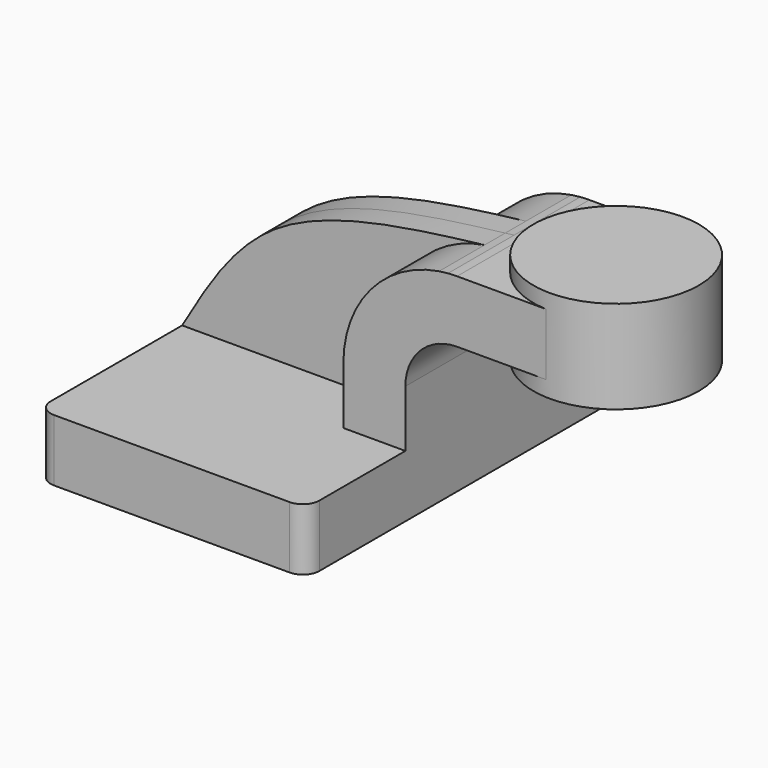
from build123d import *

# Parameters (mm, degrees)
F1_DEPTH = 63.5
F2_DEPTH = 25.4
F0_W     = 25.4
F0_H     = 19.05
F4_DEPTH = 25.4
F5_DEPTH = 7.9375
F7_R     = 5.08


# Not quite as in the source:
# - a feature names something its author has since deleted; it is built from what else it names


with BuildPart() as f1:
    # F0 (on Front) → F1 (new body, symmetric)
    with BuildSketch(Plane.XZ):
        Polygon((41.275, -9.525), (41.275, 9.525), (22.225, 9.525), (-41.275, 9.525), (-41.275, -9.525), align=None)
    extrude(amount=F1_DEPTH, both=True)

    # F0 (on Front) → F2 (join, symmetric)
    with BuildSketch(Plane.XZ):
        with BuildLine():
            Line((22.225, 9.525), (41.275, 9.525))
            Line((41.275, 9.525), (41.275, 27.0002))
            ThreePointArc((41.275, 27.0002), (45.9246798487, 38.2255201513), (57.15, 42.8752))
            Line((57.15, 42.8752), (60.325, 42.8752))
            Line((60.325, 42.8752), (60.325, 61.9252))
            Line((60.325, 61.9252), (57.15, 61.9252))
            ThreePointArc((57.15, 61.9252), (55.7573840511, 61.8974240417), (54.3669832056, 61.8141403475))
            add(Edge.make_bspline(
                [(51.6315731061, 61.4864666813), (52.5431025701, 61.5959254015), (53.4550436694, 61.7050265498), (54.3669832056, 61.8141403475)],
                knots=[0.9798743177, 0.9798743177, 0.9798743177, 0.9798743177, 1, 1, 1, 1], degree=3))
            ThreePointArc((51.6315731061, 61.4864666813), (30.5747607323, 49.6610094045), (22.225, 27.0002))
            Line((22.225, 27.0002), (22.225, 9.525))
        make_face()
    extrude(amount=F2_DEPTH, both=True)

    # F0 (on Front) → F4 (join, symmetric)
    with BuildSketch(Plane.XZ):
        with Locations((73.025, 52.4002)):
            Rectangle(F0_W, F0_H)
    extrude(amount=F4_DEPTH, both=True)

    # F0 (on Front) → F5 (join, symmetric)
    with BuildSketch(Plane.XZ):
        with BuildLine():
            Line((-41.275, 9.525), (22.225, 9.525))
            Line((22.225, 9.525), (22.225, 27.0002))
            ThreePointArc((22.225, 27.0002), (30.5747607323, 49.6610094045), (51.6315731061, 61.4864666813))
            add(Edge.make_bspline(
                [(-41.275, 9.525), (-33.3226171476, 23.2066083148), (-16.1059236769, 52.8331960278), (27.7493063598, 58.6186248213), (51.6315731061, 61.4864666813)],
                knots=[0, 0, 0, 0, 0.4525771396, 0.9798743177, 0.9798743177, 0.9798743177, 0.9798743177], degree=3))
        make_face()
    extrude(amount=F5_DEPTH, both=True)

    # F0 (on Front) → F6 (revolve)
    with BuildSketch(Plane.XZ):
        Polygon((85.725, 61.9252), (85.725, 42.8752), (85.725, 38.1), (111.125, 38.1), (111.125, 66.675), (85.725, 66.675), align=None)
    revolve(axis=Axis((85.6968834996, 0, 52.5015871972), (0, 0, -1)))

    # F7
    f7_edges = [f1.edges().sort_by_distance(p)[0] for p in [
        (41.275, -63.5, 0),
        (-41.275, -63.5, 0),
        (41.275, 63.5, 0),
        (-41.275, 63.5, 0),
    ]]
    fillet(f7_edges, radius=F7_R)


solid = f1.part
